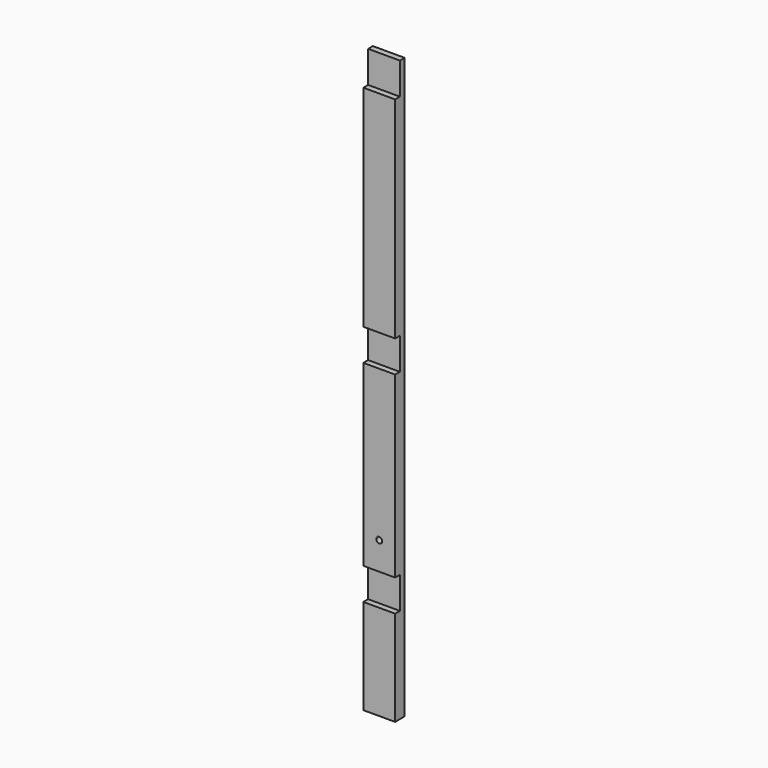
from build123d import *

# Parameters (mm, degrees)
F0_W     = 50.8
F0_H     = 19.05
F1_DEPTH = 927.1
F2_W     = 122.43557321
F2_H     = 50.8
F2_W_2   = 343.1604206562
F2_W_3   = 264.5317912102
F3_DEPTH = 25.4
F4_R     = 0.79375
F5_DEPTH = 25.4
F6_R     = 4.7625
F7_DEPTH = 25.4


# Not quite as in the source:
# - a feature names something its author has since deleted; it is built from what else it names


with BuildPart() as f1:
    # F0 (on Top) → F1 (new body)
    with BuildSketch(Plane.XY):
        Rectangle(F0_W, F0_H)
    extrude(amount=F1_DEPTH)

    # F2 (on Front) → F3 (cut)
    with BuildSketch(Plane.XZ):
        with Locations((22.4465244144, 177.8)):
            Rectangle(F2_W, F2_H)
        with Locations((-38.7818217278, 901.7)):
            Rectangle(F2_W_2, F2_H)
        with Locations((-47.6498156786, 514.35)):
            Rectangle(F2_W_3, F2_H)
    extrude(amount=F3_DEPTH, mode=Mode.SUBTRACT)

    # F4 (on Front) → F5 (cut)
    with BuildSketch(Plane.XZ):
        with Locations((9.525, 254)):
            Circle(F4_R)
        with Locations((9.525, 307.975)):
            Circle(F4_R)
        with Locations((9.525, 771.525)):
            Circle(F4_R)
        with Locations((9.525, 825.5)):
            Circle(F4_R)
        with Locations((-9.525, 771.525)):
            Circle(F4_R)
        with Locations((-9.525, 825.5)):
            Circle(F4_R)
        with Locations((-9.525, 254)):
            Circle(F4_R)
        with Locations((-9.525, 307.975)):
            Circle(F4_R)
    extrude(amount=-F5_DEPTH, mode=Mode.SUBTRACT)

    # F6 (on Front) → F7 (cut)
    with BuildSketch(Plane.XZ):
        with Locations((0, 247.65)):
            Circle(F6_R)
    extrude(amount=F7_DEPTH, mode=Mode.SUBTRACT)


solid = f1.part
